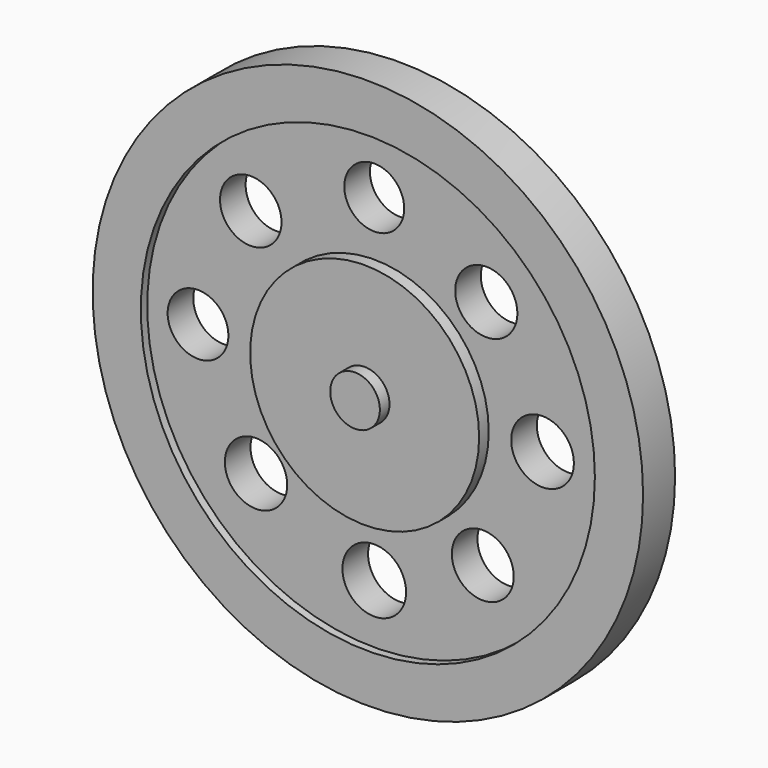
from build123d import *

# Parameters (mm, degrees)
F0_R      = 17.4625
F1_DEPTH  = 2.54
F2_R      = 14.4038068866
F3_DEPTH  = 0.508
F4_R      = 7.2639989676
F5_DEPTH  = 0.762
F6_R      = 1.5755390971
F7_DEPTH  = 0.762
F8_R      = 1.9006154527
F9_DEPTH  = 25.4
F10_R     = 2.0193
F11_DEPTH = 25.4
F12_R     = 1.927458399
F13_DEPTH = 25.4
F14_R     = 1.9885487684
F15_DEPTH = 25.4
F16_R     = 1.9516354427
F17_DEPTH = 25.4
F18_R     = 1.9777477245
F19_DEPTH = 25.4
F20_R     = 1.9643397756
F21_DEPTH = 25.4
F22_R     = 1.9730256653
F23_DEPTH = 25.4


# Not quite as in the source:
# - the program builds the solid bodies; features that only make, move or delete a surface that nothing else refers to are left out


with BuildPart() as f1:
    # F0 (on Front) → F1 (new body)
    with BuildSketch(Plane.XZ):
        Circle(F0_R)
    extrude(amount=F1_DEPTH)

    # F2 (on face) → F3 (cut)
    with BuildSketch(Plane.XZ.offset(2.54)):
        Circle(F2_R)
    extrude(amount=-F3_DEPTH, mode=Mode.SUBTRACT)

    # F4 (on face) → F5 (join)
    with BuildSketch(Plane.XZ.offset(2.032)):
        Circle(F4_R)
    extrude(amount=F5_DEPTH)

    # F6 (on face) → F7 (join)
    with BuildSketch(Plane.XZ.offset(2.794)):
        Circle(F6_R)
    extrude(amount=F7_DEPTH)

    # F8 (on face) → F9 (cut)
    with BuildSketch(Plane.XZ.offset(2.032)):
        with Locations((0, 10.7245491818)):
            Circle(F8_R)
    extrude(amount=-F9_DEPTH, mode=Mode.SUBTRACT)

    # F10 (on face) → F11 (cut)
    with BuildSketch(Plane.XZ.offset(2.032)):
        with Locations((0, -10.661974936)):
            Circle(F10_R)
    extrude(amount=-F11_DEPTH, mode=Mode.SUBTRACT)

    # F12 (on face) → F13 (cut)
    with BuildSketch(Plane.XZ.offset(2.032)):
        with Locations((-11.1813889816, 0)):
            Circle(F12_R)
    extrude(amount=-F13_DEPTH, mode=Mode.SUBTRACT)

    # F14 (on face) → F15 (cut)
    with BuildSketch(Plane.XZ.offset(2.032)):
        with Locations((10.6769250706, 0)):
            Circle(F14_R)
    extrude(amount=-F15_DEPTH, mode=Mode.SUBTRACT)

    # F16 (on face) → F17 (cut)
    with BuildSketch(Plane.XZ.offset(2.032)):
        with Locations((-7.8357290477, 7.4233920313)):
            Circle(F16_R)
    extrude(amount=-F17_DEPTH, mode=Mode.SUBTRACT)

    # F18 (on face) → F19 (cut)
    with BuildSketch(Plane.XZ.offset(2.032)):
        with Locations((-7.5011625886, -7.130230777)):
            Circle(F18_R)
    extrude(amount=-F19_DEPTH, mode=Mode.SUBTRACT)

    # F20 (on face) → F21 (cut)
    with BuildSketch(Plane.XZ.offset(2.032)):
        with Locations((6.8851769902, -7.5763189234)):
            Circle(F20_R)
    extrude(amount=-F21_DEPTH, mode=Mode.SUBTRACT)

    # F22 (on face) → F23 (cut)
    with BuildSketch(Plane.XZ.offset(2.032)):
        with Locations((7.1082208306, 7.200348191)):
            Circle(F22_R)
    extrude(amount=-F23_DEPTH, mode=Mode.SUBTRACT)


solid = f1.part
